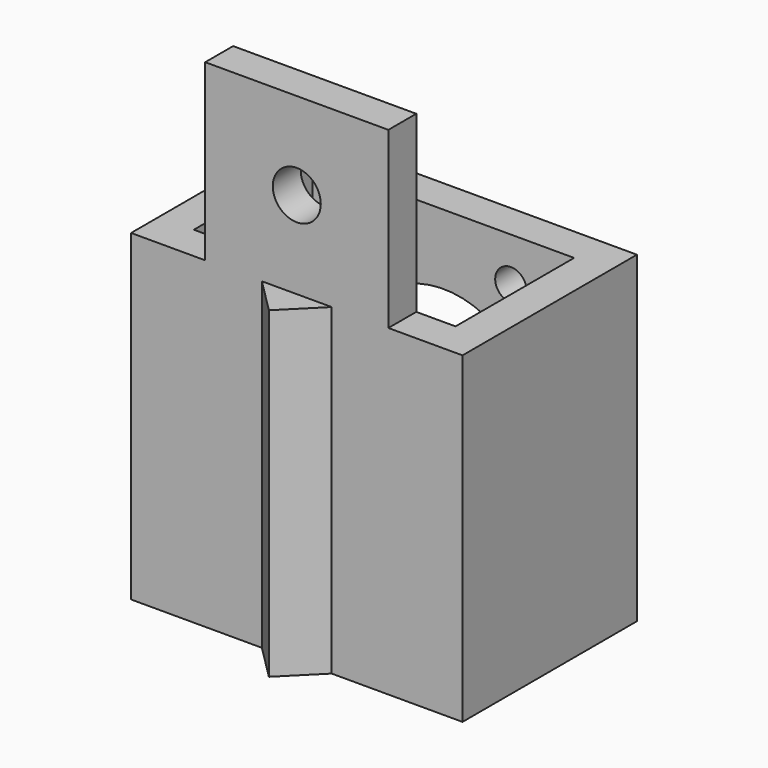
from build123d import *

# Parameters (mm, degrees)
F1_DEPTH  = 37
F3_DEPTH  = 37.001
F5_DEPTH  = 37
F7_D      = 3.6
F7_DEPTH  = 10
F7_TIP    = 1.0815491142
F8_D      = 21
F8_DEPTH  = 10
F8_TIP    = 6.3090364998
F9_W      = 11
F9_H      = 5
F10_DEPTH = 37.001
F11_W     = 21
F11_H     = 2
F12_DEPTH = 20
F14_D     = 5.5
F14_DEPTH = 12
F14_TIP   = 1.6523667023


# Not quite as in the source:
# - a feature names something its author has since deleted; it is built from what else it names


with BuildPart() as f1:
    # F0 (on Top) → F1 (new body)
    with BuildSketch(Plane.XY):
        Polygon((-13.5, 27), (-13.5, 0), (-5, 0), (5, 0), (13.5, 0), (13.5, 27), align=None)
    extrude(amount=F1_DEPTH)

    # F2 (on face) → F3 (cut, through all)
    with BuildSketch(Plane.XY.offset(37)):
        Polygon((0, 15.5), (0, 22), (-4, 26), (-10.5, 26), (-10.5, 19.5), (-6.5, 15.5), align=None)
        Polygon((4, 26), (0, 22), (0, 15.5), (6.5, 15.5), (10.5, 19.5), (10.5, 26), align=None)
        Polygon((6.5, 15.5), (0, 15.5), (0, 9), (4, 5), (10.5, 5), (10.5, 11.5), align=None)
        Polygon((0, 9), (0, 15.5), (-6.5, 15.5), (-10.5, 11.5), (-10.5, 5), (-4, 5), align=None)
        Polygon((0, 5), (0, 9), (-4, 5), align=None)
        Polygon((4, 5), (0, 9), (0, 5), align=None)
    extrude(amount=-F3_DEPTH, mode=Mode.SUBTRACT)

    # F4 (on Top) → F5 (join, through all)
    with BuildSketch(Plane.XY):
        Polygon((-13.5, 27), (0, 27), (13.5, 27), (13.5, 0), (19, 0), (19, 51), (-19, 51), (-19, 0), (-13.5, 0), align=None)
        Polygon((15, 30), (0, 30), (-15, 30), (-15, 47), (15, 47), align=None, mode=Mode.SUBTRACT)
    extrude(amount=F5_DEPTH)

    # F7
    with Locations(Plane(origin=(0, 51, 0), x_dir=(-1, 0, 0), z_dir=(0, 1, 0))):
        with Locations((-7.75, 5.0766062413), (7.75, 5.0766062413), (7.75, 31.9233937587), (-7.75, 31.9233937587)):
            Hole(F7_D / 2, depth=F7_DEPTH)
            with Locations((0, 0, -(F7_DEPTH + F7_TIP / 2))):  # 118° drill point
                Cone(0, F7_D / 2, F7_TIP, mode=Mode.SUBTRACT)

    # F8
    with Locations(Plane(origin=(0, 51, 0), x_dir=(-1, 0, 0), z_dir=(0, 1, 0))):
        with Locations((0, 18.5)):
            Hole(F8_D / 2, depth=F8_DEPTH)
            with Locations((0, 0, -(F8_DEPTH + F8_TIP / 2))):  # 118° drill point
                Cone(0, F8_D / 2, F8_TIP, mode=Mode.SUBTRACT)

    # F9 (on face) → F10 (cut, through all)
    with BuildSketch(Plane.XY.offset(37)):
        Polygon((-19, 26), (-19, 0), (-5.5, 0), (-5.5, 5), (-10.5, 5), (-10.5, 11.5), (-6.5, 15.5), (-10.5, 19.5), (-10.5, 26), align=None)
        Polygon((5.5, 5), (5.5, 0), (19, 0), (19, 26), (10.5, 26), (10.5, 19.5), (6.5, 15.5), (10.5, 11.5), (10.5, 5), align=None)
        with Locations((0, 2.5)):
            Rectangle(F9_W, F9_H)
    extrude(amount=-F10_DEPTH, mode=Mode.SUBTRACT)

    # F11 (on face) → F12 (join)
    with BuildSketch(Plane.XY.offset(37)):
        with Locations((0, 27)):
            Rectangle(F11_W, F11_H)
        with Locations((0, 29)):
            Rectangle(F11_W, F11_H)
        Polygon((4, 26), (10.5, 26), (10.5, 28), (-10.5, 28), (-10.5, 26), (-4, 26), align=None)
    extrude(amount=F12_DEPTH)

    # F14
    with Locations(Plane(origin=(0, 30, 0), x_dir=(-1, 0, 0), z_dir=(0, 1, 0))):
        with Locations((0, 47)):
            Hole(F14_D / 2, depth=F14_DEPTH)
            with Locations((0, 0, -(F14_DEPTH + F14_TIP / 2))):  # 118° drill point
                Cone(0, F14_D / 2, F14_TIP, mode=Mode.SUBTRACT)


solid = f1.part
